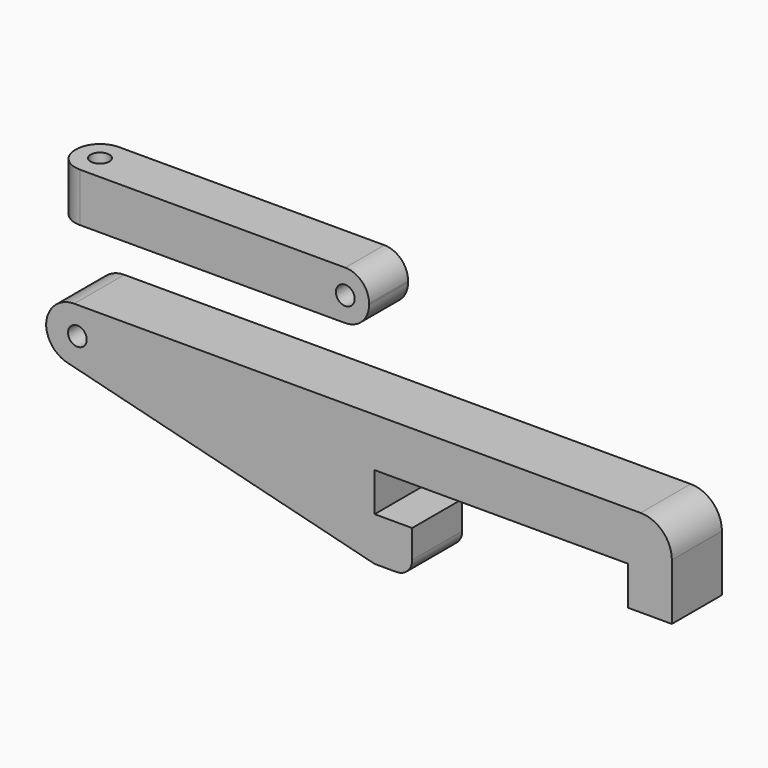
from build123d import *

# Parameters (mm, degrees)
F1_DEPTH    = 10
F2_R        = 5
F3_R        = 2.5
F4_T1_DEPTH = 27.5431430313
F4_T3_DEPTH = 32.5
F5_R        = 1.5
F6_DEPTH    = 25
F7_W        = 50
F7_H        = 7.8
F7_R        = 1.5
F8_DEPTH    = 7.8
F9_R        = 3.8
F10_R       = 1.5
F11_DEPTH   = 25


# Not quite as in the source:
# - a fillet or chamfer that OpenCascade refuses, or shapes differently, is made with other operations: its cross-section is extruded or revolved along the edge and cut away or added


with BuildPart() as f1:
    # F0 (on Front) → F1 (new body)
    with BuildSketch(Plane.XZ):
        Polygon((-40.5, 0), (0, 0), (0, -6.2), (7, -6.2), (7, 7.8), (-93, 7.8), (-93, 0), (-40.5, -13.2), (-34.5, -13.2), (-34.5, -6.2), (-40.5, -6.2), align=None)
    extrude(amount=F1_DEPTH)

    # F2
    f2_edges = [f1.edges().sort_by_distance(p)[0] for p in [
        (7, -5, 7.8),
    ]]
    fillet(f2_edges, radius=F2_R)

    # F3
    f3_edges = [f1.edges().sort_by_distance(p)[0] for p in [
        (-34.5, -5, -13.2),
        (-40.5, -5, -13.2),
    ]]
    fillet(f3_edges, radius=F3_R)

    # F4: fillet of radius 4.5 on 2 edges, made by hand

    # F4_s2 → F4_t1 (cut)
    with BuildSketch(Plane.XZ.offset(-8.7715715157)):
        with BuildLine():
            ThreePointArc((-89.5972771189, -0.855541753), (-92.0487847945, 0.7416579735), (-93, 3.5086286063))
            Line((-93, 3.5086286063), (-93, 0))
            Line((-93, 0), (-89.5972771189, -0.855541753))
        make_face()
    extrude(amount=F4_T1_DEPTH, mode=Mode.SUBTRACT)

    # F4_s4 → F4_t3 (cut)
    with BuildSketch(Plane.XZ.offset(-11.25)):
        with BuildLine():
            ThreePointArc((-93, 3.3), (-91.6819805153, 6.4819805153), (-88.5, 7.8))
            Line((-88.5, 7.8), (-93, 7.8))
            Line((-93, 7.8), (-93, 3.3))
        make_face()
    extrude(amount=F4_T3_DEPTH, mode=Mode.SUBTRACT)

    # F5 (on face) → F6 (cut)
    with BuildSketch(Plane.XZ.offset(10)):
        with Locations((-88, 3.4)):
            Circle(F5_R)
    extrude(amount=-F6_DEPTH, mode=Mode.SUBTRACT)


with BuildPart() as f8:
    # F7 (on Front) → F8 (new body)
    with BuildSketch(Plane.XZ):
        with Locations((-68.1472382043, 21.5872781662)):
            Rectangle(F7_W, F7_H)
        with Locations((-46.9472382043, 21.5872781662)):
            Circle(F7_R, mode=Mode.SUBTRACT)
    extrude(amount=F8_DEPTH)

    # F9
    f9_edges = [f8.edges().sort_by_distance(p)[0] for p in [
        (-43.147238, -3.9, 25.487278),
        (-43.147238, -3.9, 17.687278),
        (-93.147238, -7.8, 21.587278),
        (-93.147238, 0, 21.587278),
    ]]
    fillet(f9_edges, radius=F9_R)

    # F10 (on face) → F11 (cut)
    with BuildSketch(Plane.XY.offset(25.4872781662)):
        with Locations((-89.3472382043, -3.8)):
            Circle(F10_R)
    extrude(amount=-F11_DEPTH, mode=Mode.SUBTRACT)


solid = Compound([f1.part, f8.part])
